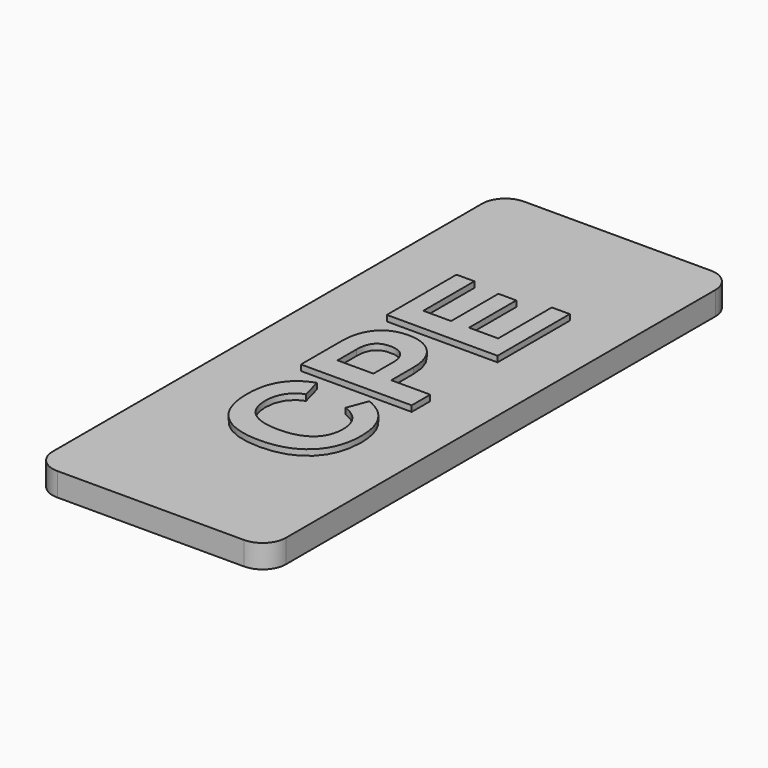
from build123d import *

# Parameters (mm, degrees)
F0_W         = 20
F0_H         = 50
F1_DEPTH     = 2
F2_R         = 2
F3_TEXT_SIZE = 13.7895914829
F4_DEPTH     = 2.5


# Not quite as in the source:
# - Text() gives the source's letters only with a copy of the font that has no kerning and outlines rounded to 1/6400 em; it was checked with that copy


with BuildPart() as f1:
    # F0 (on Top) → F1 (new body)
    with BuildSketch(Plane.XY):
        with Locations((-10, 0)):
            Rectangle(F0_W, F0_H)
    extrude(amount=F1_DEPTH)

    # F2
    f2_edges = [f1.edges().sort_by_distance(p)[0] for p in [
        (0, -25, 1),
        (-20, -25, 1),
        (0, 25, 1),
        (-20, 25, 1),
    ]]
    fillet(f2_edges, radius=F2_R)


with BuildPart() as f4:
    # F3 (on Top) → F4 (new body)
    with BuildSketch(Plane.XY):
        with Locations(Location((-4.823861178, -14.3864222393), (0, 0, 90))):
            Text('CPE', F3_TEXT_SIZE, font='Arimo', font_style=FontStyle.BOLD, text_align=(TextAlign.LEFT, TextAlign.BOTTOM))
    extrude(amount=F4_DEPTH)


solid = Compound([f1.part, f4.part])
